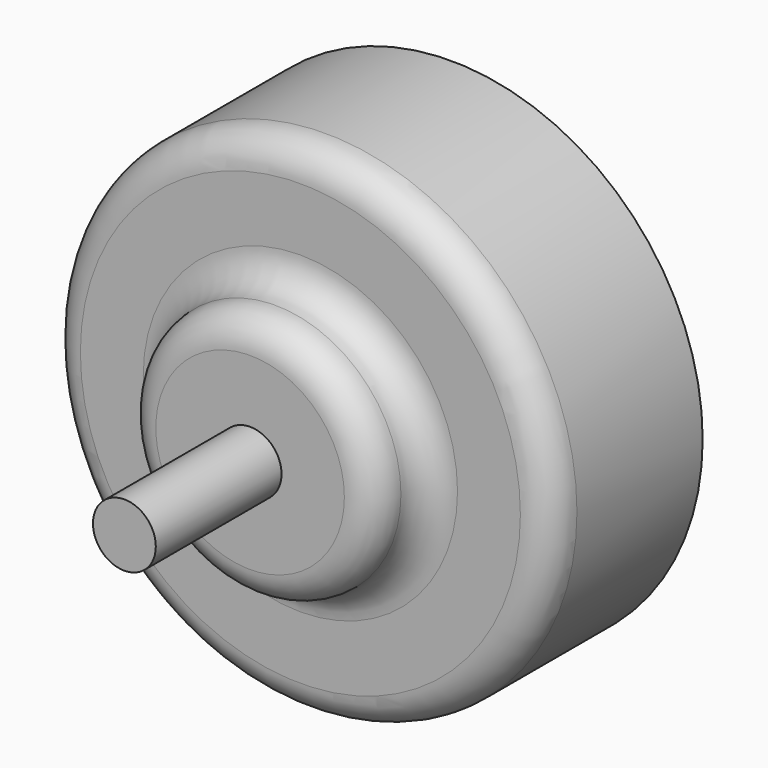
from build123d import *

# Parameters (mm, degrees)
F0_R     = 40
F0_R_2   = 30
F1_DEPTH = 20
F2_R     = 40
F2_R_2   = 30
F3_DEPTH = 10
F4_R     = 20
F5_DEPTH = 10
F6_R     = 5
F7_DEPTH = 25
F8_R     = 4.99999
F9_R     = 5


# Not quite as in the source:
# - a fillet or chamfer is up to 0.001 mm smaller than in the source, because OpenCascade refuses the exact size


with BuildPart() as f1:
    # F0 (on Front) → F1 (new body)
    with BuildSketch(Plane.XZ):
        Circle(F0_R)
        Circle(F0_R_2, mode=Mode.SUBTRACT)
    extrude(amount=F1_DEPTH)

    # F2 (on face) → F3 (join)
    with BuildSketch(Plane.XZ.offset(20)):
        Circle(F2_R)
        Circle(F2_R_2, mode=Mode.SUBTRACT)
        Circle(F2_R_2)
    extrude(amount=F3_DEPTH)

    # F4 (on face) → F5 (join)
    with BuildSketch(Plane.XZ.offset(30)):
        Circle(F4_R)
    extrude(amount=F5_DEPTH)

    # F6 (on face) → F7 (join)
    with BuildSketch(Plane.XZ.offset(40)):
        Circle(F6_R)
    extrude(amount=F7_DEPTH)

    # F8 (radius 5 in the source; OpenCascade refuses exactly that, so slightly less here)
    f8_edges = [f1.edges().sort_by_distance(p)[0] for p in [
        (-20, -30, 0),
        (-20, -40, 0),
    ]]
    fillet(f8_edges, radius=F8_R)

    # F9
    f9_edges = [f1.edges().sort_by_distance(p)[0] for p in [
        (-40, -30, 0),
    ]]
    fillet(f9_edges, radius=F9_R)


solid = f1.part
